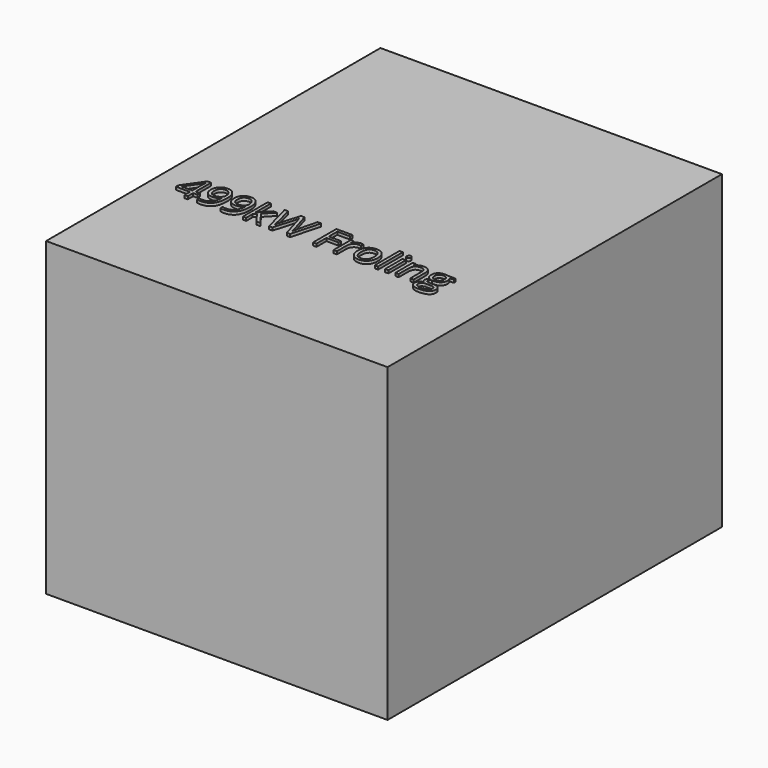
from build123d import *

# Parameters (mm, degrees)
F0_W         = 2990
F0_H         = 3660
F1_DEPTH     = 2720
F2_TEXT_SIZE = 356.3777440124
F3_DEPTH     = 25


# Not quite as in the source:
# - Text() gives the source's letters only with a copy of the font that has no kerning and outlines rounded to 1/6400 em; it was checked with that copy


with BuildPart() as f1:
    # F0 (on Top) → F1 (new body)
    with BuildSketch(Plane.XY):
        with Locations((1495, 1830)):
            Rectangle(F0_W, F0_H)
    extrude(amount=F1_DEPTH)

    # F2 (on face) → F3 (join)
    with BuildSketch(Plane.XY.offset(2720)):
        with Locations((212.6644253731, 1086.6961479187)):
            Text('499kW Froling', F2_TEXT_SIZE, font='Open Sans', text_align=(TextAlign.LEFT, TextAlign.BOTTOM))
    extrude(amount=F3_DEPTH)


solid = f1.part
